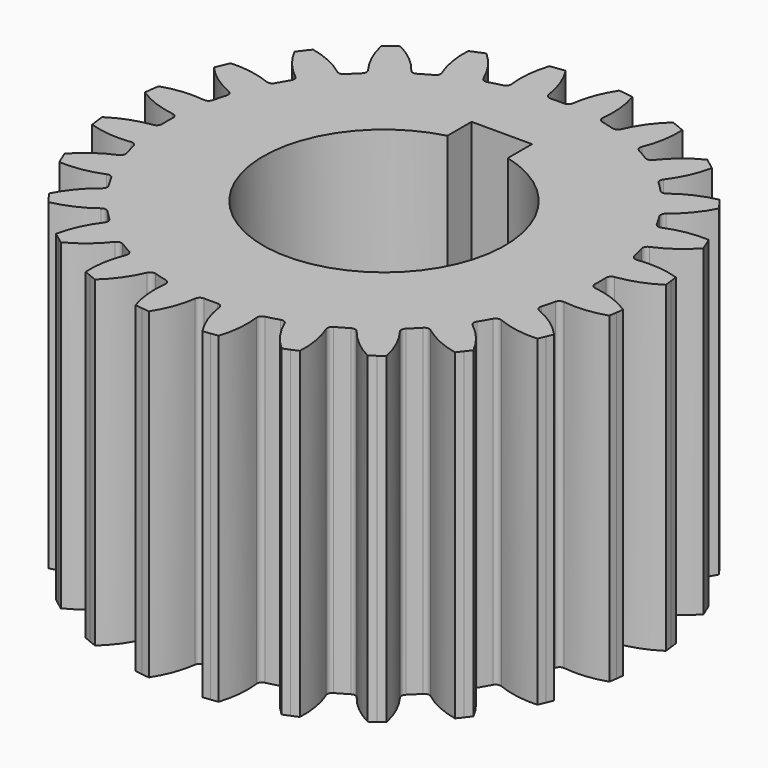
from build123d import *

# Parameters (mm, degrees)
F0_R            = 17.0688
F1_DEPTH        = 25.4
F3_DEPTH        = 25.401
F5_DEPTH        = 25.4
F5_COPIES_COUNT = 24
F6_R            = 0.4064


# Not quite as in the source:
# - a pattern or mirror of a feature is missing from the dataset's text; its kind, count and spacing are read off the source's solid


with BuildPart() as f1:
    # F0 (on Top) → F1 (new body)
    with BuildSketch(Plane.XY):
        Circle(F0_R)
    extrude(amount=F1_DEPTH)

    # F2 (on face) → F3 (cut, through all)
    with BuildSketch(Plane.XY.offset(25.4)):
        with BuildLine():
            Line((-2.38125, 11.6037915932), (-2.38125, 9.2225415932))
            ThreePointArc((-2.38125, 9.2225415932), (0, -9.525), (2.38125, 9.2225415932))
            Line((2.38125, 9.2225415932), (2.38125, 11.6037915932))
            Line((2.38125, 11.6037915932), (-2.38125, 11.6037915932))
        make_face()
    extrude(amount=-F3_DEPTH, mode=Mode.SUBTRACT)

    # F4 (on face) → F5 (join, through all)
    with BuildSketch(Plane.XY.offset(25.4)):
        with BuildLine():
            ThreePointArc((-3.5361735829, 16.6984852556), (-2.2279254698, 16.9227740498), (-0.9062046185, 17.0447272383))
            ThreePointArc((-0.9062046185, 17.0447272383), (-1.2948406344, 18.8609591508), (-2.1113315127, 20.5292154135))
            ThreePointArc((-2.1113315127, 20.5292154135), (-2.4027753986, 20.4971480122), (-2.6937342919, 20.4609433266))
            ThreePointArc((-2.6937342919, 20.4609433266), (-2.9841494635, 20.4206086645), (-3.273962294, 20.3761521674))
            ThreePointArc((-3.273962294, 20.3761521674), (-3.6308554274, 18.5534169689), (-3.5361735829, 16.6984852556))
        make_face()
    f5 = extrude(amount=-F5_DEPTH)

    # F5_copies: F5 ×24 about axis
    f5_copies_axis = Axis((0, 0, 0), (0, 0, 1))
    for i in range(1, F5_COPIES_COUNT):
        add(f5.rotate(f5_copies_axis, i * 360 / F5_COPIES_COUNT))

    # F6
    f6_edges = [f1.edges().sort_by_distance(p)[0] for p in [
        (-0.906205, 17.044727, 12.7),
        (-3.536174, 16.698485, 12.7),
        (-9.30716, 14.308064, 12.7),
        (-7.737567, 15.214269, 12.7),
        (-5.286826, 16.229399, 12.7),
        (-11.411659, 12.693226, 12.7),
        (-12.693226, 11.411659, 12.7),
        (-14.308064, 9.30716, 12.7),
        (-15.214269, 7.737567, 12.7),
        (-16.229399, 5.286826, 12.7),
        (-16.698485, 3.536174, 12.7),
        (-17.044727, 0.906205, 12.7),
        (-17.044727, -0.906205, 12.7),
        (-16.698485, -3.536174, 12.7),
        (-16.229399, -5.286826, 12.7),
        (-15.214269, -7.737567, 12.7),
        (-14.308064, -9.30716, 12.7),
        (-12.693226, -11.411659, 12.7),
        (-11.411659, -12.693226, 12.7),
        (-9.30716, -14.308064, 12.7),
        (-7.737567, -15.214269, 12.7),
        (-5.286826, -16.229399, 12.7),
        (-3.536174, -16.698485, 12.7),
        (-0.906205, -17.044727, 12.7),
        (0.906205, -17.044727, 12.7),
        (3.536174, -16.698485, 12.7),
        (5.286826, -16.229399, 12.7),
        (7.737567, -15.214269, 12.7),
        (9.30716, -14.308064, 12.7),
        (11.411659, -12.693226, 12.7),
        (12.693226, -11.411659, 12.7),
        (14.308064, -9.30716, 12.7),
        (15.214269, -7.737567, 12.7),
        (16.229399, -5.286826, 12.7),
        (16.698485, -3.536174, 12.7),
        (17.044727, -0.906205, 12.7),
        (17.044727, 0.906205, 12.7),
        (16.698485, 3.536174, 12.7),
        (16.229399, 5.286826, 12.7),
        (15.214269, 7.737567, 12.7),
        (14.308064, 9.30716, 12.7),
        (12.693226, 11.411659, 12.7),
        (11.411659, 12.693226, 12.7),
        (9.30716, 14.308064, 12.7),
        (7.737567, 15.214269, 12.7),
        (5.286826, 16.229399, 12.7),
        (3.536174, 16.698485, 12.7),
        (0.906205, 17.044727, 12.7),
    ]]
    fillet(f6_edges, radius=F6_R)


solid = f1.part
